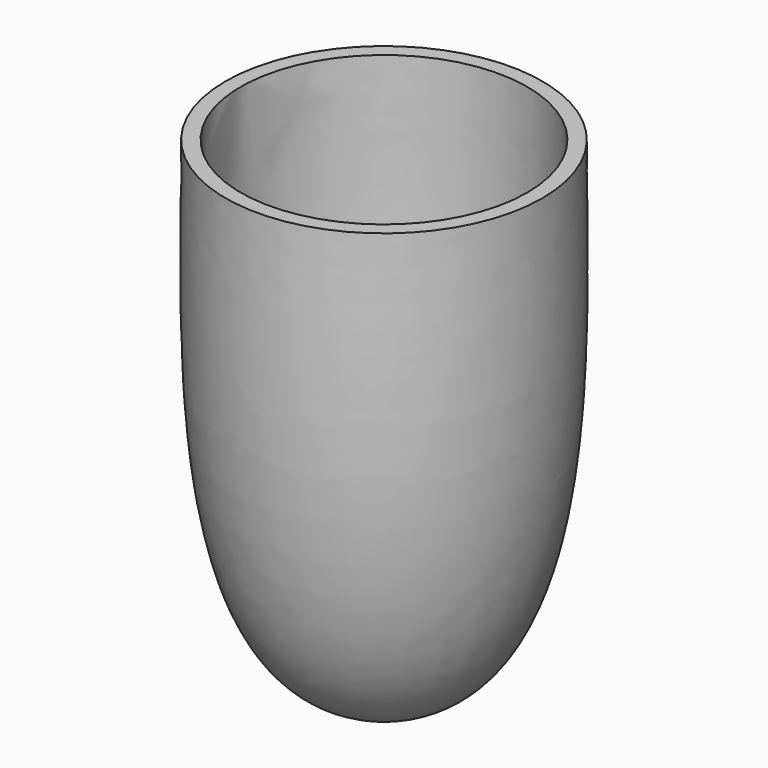
from build123d import *


# Not quite as in the source:
# - the dataset's text gives a spline's control points without its knots; the knots are read off the source's solid


with BuildPart() as f1:
    # F0 (on Front) → F1 (revolve)
    with BuildSketch(Plane.XZ):
        with BuildLine():
            Line((0, 2), (0, 0))
            add(Edge.make_bspline(
                [(0, 0), (23.5498647262, 0), (20.9320783615, 41.7081862688), (20.9320783615, 65.5831545591)],
                knots=[0, 0, 0, 0, 68.8425890453, 68.8425890453, 68.8425890453, 68.8425890453], degree=3))
            Line((20.9320783615, 65.5831545591), (18.9320783615, 65.5831545591))
            add(Edge.make_bspline(
                [(0, 2), (1.3242783435, 2), (3.7384264007, 2.2923115555), (6.7774530121, 3.4795618758), (9.3823646779, 5.3633768045), (11.6355334339, 7.9431458318), (13.5525171646, 11.1889476515), (15.6648362966, 16.3093300516), (17.5020628605, 23.9677952847), (18.6488827554, 34.4011235836), (19.0444021256, 45.3335690122), (19.014059508, 56.0481279708), (18.9320783615, 62.5805092482), (18.9320783615, 65.5831545591)],
                knots=[0, 0, 0, 0, 0.0625, 0.125, 0.1875, 0.25, 0.3125, 0.375, 0.5, 0.625, 0.75, 0.875, 1, 1, 1, 1], degree=3))
        make_face()
    revolve(axis=Axis((0, 0, 1), (0, 0, -1)))


solid = f1.part
